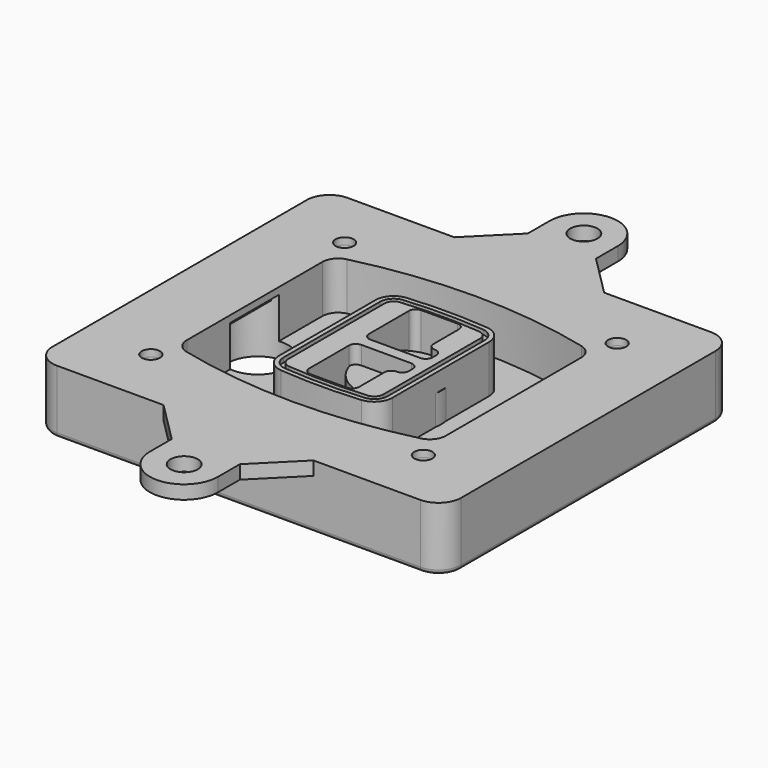
from build123d import *

# Parameters (mm, degrees)
F0_R      = 4
F1_DEPTH  = 25
F2_DEPTH  = 3
F3_DEPTH  = 18
F5_DEPTH  = 21
F6_DEPTH  = 2
F8_DEPTH  = 20
F9_DEPTH  = 16
F10_DEPTH = 25
F7_R      = 6
F7_R_2    = 4
F11_DEPTH = 6
F13_DEPTH = 9
F15_R     = 2
F16_R     = 4
F16_R_2   = 6
F17_DEPTH = 3


# Not quite as in the source:
# - a feature of the source that left no trace in its solid (it failed there, or was rolled back) is left out
# - a feature names something its author has since deleted; it is built from what else it names


with BuildPart() as f1:
    # F0 (on Top) → F1 (new body)
    with BuildSketch(Plane.XY):
        with BuildLine():
            ThreePointArc((-90, -70), (-87.0710678119, -77.0710678119), (-80, -80))
            Line((-80, -80), (80, -80))
            ThreePointArc((80, -80), (87.0710678119, -77.0710678119), (90, -70))
            Line((90, -70), (90, 70))
            ThreePointArc((90, 70), (87.0710678119, 77.0710678119), (80, 80))
            Line((80, 80), (-80, 80))
            ThreePointArc((-80, 80), (-87.0710678119, 77.0710678119), (-90, 70))
            Line((-90, 70), (-90, -70))
        make_face()
        with Locations((-60, -53.3333333333)):
            Circle(F0_R, mode=Mode.SUBTRACT)
        with Locations((60, -53.3333333333)):
            Circle(F0_R, mode=Mode.SUBTRACT)
        with Locations((-60, 53.3333333333)):
            Circle(F0_R, mode=Mode.SUBTRACT)
        with BuildLine():
            ThreePointArc((-64, 37.2990447398), (-61.0143011354, 45.9411029726), (-53.3306899286, 50.8970778549))
            ThreePointArc((-53.3306899286, 50.8970778549), (0, 57.3333333333), (53.3306899286, 50.8970778549))
            ThreePointArc((53.3306899286, 50.8970778549), (61.0143011354, 45.9411029726), (64, 37.2990447398))
            Line((64, 37.2990447398), (64, -37.2990447398))
            ThreePointArc((64, -37.2990447398), (61.0143011354, -45.9411029726), (53.3306899286, -50.8970778549))
            ThreePointArc((53.3306899286, -50.8970778549), (0, -57.3333333333), (-53.3306899286, -50.8970778549))
            ThreePointArc((-53.3306899286, -50.8970778549), (-61.0143011354, -45.9411029726), (-64, -37.2990447398))
            Line((-64, -37.2990447398), (-64, 37.2990447398))
        make_face(mode=Mode.SUBTRACT)
        with Locations((60, 53.3333333333)):
            Circle(F0_R, mode=Mode.SUBTRACT)
        with BuildLine():
            ThreePointArc((53.3306899286, 50.8970778549), (0, 57.3333333333), (-53.3306899286, 50.8970778549))
            ThreePointArc((-53.3306899286, 50.8970778549), (-61.0143011354, 45.9411029726), (-64, 37.2990447398))
            Line((-64, 37.2990447398), (-64, -37.2990447398))
            ThreePointArc((-64, -37.2990447398), (-61.0143011354, -45.9411029726), (-53.3306899286, -50.8970778549))
            ThreePointArc((-53.3306899286, -50.8970778549), (0, -57.3333333333), (53.3306899286, -50.8970778549))
            ThreePointArc((53.3306899286, -50.8970778549), (61.0143011354, -45.9411029726), (64, -37.2990447398))
            Line((64, -37.2990447398), (64, 37.2990447398))
            ThreePointArc((64, 37.2990447398), (61.0143011354, 45.9411029726), (53.3306899286, 50.8970778549))
        make_face()
        with BuildLine():
            Line((-60, -37.2990447398), (-60, 37.2990447398))
            ThreePointArc((-60, 37.2990447398), (-57.8673579538, 43.4719434775), (-52.3790642347, 47.0119255363))
            ThreePointArc((-52.3790642347, 47.0119255363), (0, 53.3333333333), (52.3790642347, 47.0119255363))
            ThreePointArc((52.3790642347, 47.0119255363), (57.8673579538, 43.4719434775), (60, 37.2990447398))
            Line((60, 37.2990447398), (60, -37.2990447398))
            ThreePointArc((60, -37.2990447398), (57.8673579538, -43.4719434775), (52.3790642347, -47.0119255363))
            ThreePointArc((52.3790642347, -47.0119255363), (0, -53.3333333333), (-52.3790642347, -47.0119255363))
            ThreePointArc((-52.3790642347, -47.0119255363), (-57.8673579538, -43.4719434775), (-60, -37.2990447398))
        make_face(mode=Mode.SUBTRACT)
        with BuildLine():
            ThreePointArc((-52.3790642347, 47.0119255363), (-57.8673579538, 43.4719434775), (-60, 37.2990447398))
            Line((-60, 37.2990447398), (-60, -37.2990447398))
            ThreePointArc((-60, -37.2990447398), (-57.8673579538, -43.4719434775), (-52.3790642347, -47.0119255363))
            ThreePointArc((-52.3790642347, -47.0119255363), (0, -53.3333333333), (52.3790642347, -47.0119255363))
            ThreePointArc((52.3790642347, -47.0119255363), (57.8673579538, -43.4719434775), (60, -37.2990447398))
            Line((60, -37.2990447398), (60, 37.2990447398))
            ThreePointArc((60, 37.2990447398), (57.8673579538, 43.4719434775), (52.3790642347, 47.0119255363))
            ThreePointArc((52.3790642347, 47.0119255363), (0, 53.3333333333), (-52.3790642347, 47.0119255363))
        make_face()
        with BuildLine():
            ThreePointArc((51.6653449643, 44.0980612973), (55.5071505677, 41.6200738562), (57, 37.2990447398))
            Line((57, 37.2990447398), (57, -37.2990447398))
            ThreePointArc((57, -37.2990447398), (55.5071505677, -41.6200738562), (51.6653449643, -44.0980612973))
            ThreePointArc((51.6653449643, -44.0980612973), (0, -50.3333333333), (-51.6653449643, -44.0980612973))
            ThreePointArc((-51.6653449643, -44.0980612973), (-55.5071505677, -41.6200738562), (-57, -37.2990447398))
            Line((-57, -37.2990447398), (-57, 37.2990447398))
            ThreePointArc((-57, 37.2990447398), (-55.5071505677, 41.6200738562), (-51.6653449643, 44.0980612973))
            ThreePointArc((-51.6653449643, 44.0980612973), (0, 50.3333333333), (51.6653449643, 44.0980612973))
        make_face(mode=Mode.SUBTRACT)
        with BuildLine():
            Line((57, -37.2990447398), (57, 37.2990447398))
            ThreePointArc((57, 37.2990447398), (55.5071505677, 41.6200738562), (51.6653449643, 44.0980612973))
            ThreePointArc((51.6653449643, 44.0980612973), (0, 50.3333333333), (-51.6653449643, 44.0980612973))
            ThreePointArc((-51.6653449643, 44.0980612973), (-55.5071505677, 41.6200738562), (-57, 37.2990447398))
            Line((-57, 37.2990447398), (-57, -37.2990447398))
            ThreePointArc((-57, -37.2990447398), (-55.5071505677, -41.6200738562), (-51.6653449643, -44.0980612973))
            ThreePointArc((-51.6653449643, -44.0980612973), (0, -50.3333333333), (51.6653449643, -44.0980612973))
            ThreePointArc((51.6653449643, -44.0980612973), (55.5071505677, -41.6200738562), (57, -37.2990447398))
        make_face()
    extrude(amount=-F1_DEPTH)

    # F0 (on Top) → F2 (join)
    with BuildSketch(Plane.XY):
        with BuildLine():
            ThreePointArc((-52.3790642347, 47.0119255363), (-57.8673579538, 43.4719434775), (-60, 37.2990447398))
            Line((-60, 37.2990447398), (-60, -37.2990447398))
            ThreePointArc((-60, -37.2990447398), (-57.8673579538, -43.4719434775), (-52.3790642347, -47.0119255363))
            ThreePointArc((-52.3790642347, -47.0119255363), (0, -53.3333333333), (52.3790642347, -47.0119255363))
            ThreePointArc((52.3790642347, -47.0119255363), (57.8673579538, -43.4719434775), (60, -37.2990447398))
            Line((60, -37.2990447398), (60, 37.2990447398))
            ThreePointArc((60, 37.2990447398), (57.8673579538, 43.4719434775), (52.3790642347, 47.0119255363))
            ThreePointArc((52.3790642347, 47.0119255363), (0, 53.3333333333), (-52.3790642347, 47.0119255363))
        make_face()
        with BuildLine():
            ThreePointArc((51.6653449643, 44.0980612973), (55.5071505677, 41.6200738562), (57, 37.2990447398))
            Line((57, 37.2990447398), (57, -37.2990447398))
            ThreePointArc((57, -37.2990447398), (55.5071505677, -41.6200738562), (51.6653449643, -44.0980612973))
            ThreePointArc((51.6653449643, -44.0980612973), (0, -50.3333333333), (-51.6653449643, -44.0980612973))
            ThreePointArc((-51.6653449643, -44.0980612973), (-55.5071505677, -41.6200738562), (-57, -37.2990447398))
            Line((-57, -37.2990447398), (-57, 37.2990447398))
            ThreePointArc((-57, 37.2990447398), (-55.5071505677, 41.6200738562), (-51.6653449643, 44.0980612973))
            ThreePointArc((-51.6653449643, 44.0980612973), (0, 50.3333333333), (51.6653449643, 44.0980612973))
        make_face(mode=Mode.SUBTRACT)
    extrude(amount=F2_DEPTH)

    # F0 (on Top) → F3 (cut)
    with BuildSketch(Plane.XY):
        with BuildLine():
            Line((57, -37.2990447398), (57, 37.2990447398))
            ThreePointArc((57, 37.2990447398), (55.5071505677, 41.6200738562), (51.6653449643, 44.0980612973))
            ThreePointArc((51.6653449643, 44.0980612973), (0, 50.3333333333), (-51.6653449643, 44.0980612973))
            ThreePointArc((-51.6653449643, 44.0980612973), (-55.5071505677, 41.6200738562), (-57, 37.2990447398))
            Line((-57, 37.2990447398), (-57, -37.2990447398))
            ThreePointArc((-57, -37.2990447398), (-55.5071505677, -41.6200738562), (-51.6653449643, -44.0980612973))
            ThreePointArc((-51.6653449643, -44.0980612973), (0, -50.3333333333), (51.6653449643, -44.0980612973))
            ThreePointArc((51.6653449643, -44.0980612973), (55.5071505677, -41.6200738562), (57, -37.2990447398))
        make_face()
    extrude(amount=-F3_DEPTH, mode=Mode.SUBTRACT)

    # F4 (on face) → F5 (join, through all)
    with BuildSketch(Plane.XY.offset(3)):
        with BuildLine():
            ThreePointArc((-25, -26.587695628), (-22.8992979869, -31.9912392117), (-17.7004291845, -34.5569740744))
            ThreePointArc((-17.7004291845, -34.5569740744), (0, -35.3333333333), (17.7004291845, -34.5569740744))
            ThreePointArc((17.7004291845, -34.5569740744), (22.8992979869, -31.9912392117), (25, -26.587695628))
            Line((25, -26.587695628), (25, 26.587695628))
            ThreePointArc((25, 26.587695628), (22.8992979869, 31.9912392117), (17.7004291845, 34.5569740744))
            ThreePointArc((17.7004291845, 34.5569740744), (0, 35.3333333333), (-17.7004291845, 34.5569740744))
            ThreePointArc((-17.7004291845, 34.5569740744), (-22.8992979869, 31.9912392117), (-25, 26.587695628))
            Line((-25, 26.587695628), (-25, -26.587695628))
        make_face()
        with BuildLine():
            ThreePointArc((17.5253218884, 32.5646544628), (21.4244734902, 30.6403533158), (23, 26.587695628))
            Line((23, 26.587695628), (23, -26.587695628))
            ThreePointArc((23, -26.587695628), (21.4244734902, -30.6403533158), (17.5253218884, -32.5646544628))
            ThreePointArc((17.5253218884, -32.5646544628), (0, -33.3333333333), (-17.5253218884, -32.5646544628))
            ThreePointArc((-17.5253218884, -32.5646544628), (-21.4244734902, -30.6403533158), (-23, -26.587695628))
            Line((-23, -26.587695628), (-23, 26.587695628))
            ThreePointArc((-23, 26.587695628), (-21.4244734902, 30.6403533158), (-17.5253218884, 32.5646544628))
            ThreePointArc((-17.5253218884, 32.5646544628), (0, 33.3333333333), (17.5253218884, 32.5646544628))
        make_face(mode=Mode.SUBTRACT)
        with BuildLine():
            Line((23, -26.587695628), (23, 26.587695628))
            ThreePointArc((23, 26.587695628), (21.4244734902, 30.6403533158), (17.5253218884, 32.5646544628))
            ThreePointArc((17.5253218884, 32.5646544628), (0, 33.3333333333), (-17.5253218884, 32.5646544628))
            ThreePointArc((-17.5253218884, 32.5646544628), (-21.4244734902, 30.6403533158), (-23, 26.587695628))
            Line((-23, 26.587695628), (-23, -26.587695628))
            ThreePointArc((-23, -26.587695628), (-21.4244734902, -30.6403533158), (-17.5253218884, -32.5646544628))
            ThreePointArc((-17.5253218884, -32.5646544628), (0, -33.3333333333), (17.5253218884, -32.5646544628))
            ThreePointArc((17.5253218884, -32.5646544628), (21.4244734902, -30.6403533158), (23, -26.587695628))
        make_face()
        with BuildLine():
            ThreePointArc((17.3502145923, 30.5723348512), (19.9496489934, 29.2894674198), (21, 26.587695628))
            Line((21, 26.587695628), (21, -26.587695628))
            ThreePointArc((21, -26.587695628), (19.9496489934, -29.2894674198), (17.3502145923, -30.5723348512))
            ThreePointArc((17.3502145923, -30.5723348512), (0, -31.3333333333), (-17.3502145923, -30.5723348512))
            ThreePointArc((-17.3502145923, -30.5723348512), (-19.9496489934, -29.2894674198), (-21, -26.587695628))
            Line((-21, -26.587695628), (-21, 26.587695628))
            ThreePointArc((-21, 26.587695628), (-19.9496489934, 29.2894674198), (-17.3502145923, 30.5723348512))
            ThreePointArc((-17.3502145923, 30.5723348512), (0, 31.3333333333), (17.3502145923, 30.5723348512))
        make_face(mode=Mode.SUBTRACT)
        with BuildLine():
            Line((21, -26.587695628), (21, 26.587695628))
            ThreePointArc((21, 26.587695628), (19.9496489934, 29.2894674198), (17.3502145923, 30.5723348512))
            ThreePointArc((17.3502145923, 30.5723348512), (0, 31.3333333333), (-17.3502145923, 30.5723348512))
            ThreePointArc((-17.3502145923, 30.5723348512), (-19.9496489934, 29.2894674198), (-21, 26.587695628))
            Line((-21, 26.587695628), (-21, -26.587695628))
            ThreePointArc((-21, -26.587695628), (-19.9496489934, -29.2894674198), (-17.3502145923, -30.5723348512))
            ThreePointArc((-17.3502145923, -30.5723348512), (0, -31.3333333333), (17.3502145923, -30.5723348512))
            ThreePointArc((17.3502145923, -30.5723348512), (19.9496489934, -29.2894674198), (21, -26.587695628))
        make_face()
        with BuildLine():
            Line((-8, -2.5), (14, -2.5))
            ThreePointArc((14, -2.5), (16.1213203436, -3.3786796564), (17, -5.5))
            Line((17, -5.5), (17, -7.5))
            ThreePointArc((17, -7.5), (16.1213203436, -9.6213203436), (14, -10.5))
            ThreePointArc((14, -10.5), (11.8786796564, -11.3786796564), (11, -13.5))
            Line((11, -13.5), (11, -27.5))
            ThreePointArc((11, -27.5), (10.1213203436, -29.6213203436), (8, -30.5))
            Line((8, -30.5), (-8, -30.5))
            ThreePointArc((-8, -30.5), (-10.1213203436, -29.6213203436), (-11, -27.5))
            Line((-11, -27.5), (-11, -5.5))
            ThreePointArc((-11, -5.5), (-10.1213203436, -3.3786796564), (-8, -2.5))
        make_face(mode=Mode.SUBTRACT)
        with BuildLine():
            ThreePointArc((-8, 2.5), (-10.1213203436, 3.3786796564), (-11, 5.5))
            Line((-11, 5.5), (-11, 27.5))
            ThreePointArc((-11, 27.5), (-10.1213203436, 29.6213203436), (-8, 30.5))
            Line((-8, 30.5), (8, 30.5))
            ThreePointArc((8, 30.5), (10.1213203436, 29.6213203436), (11, 27.5))
            Line((11, 27.5), (11, 13.5))
            ThreePointArc((11, 13.5), (11.8786796564, 11.3786796564), (14, 10.5))
            ThreePointArc((14, 10.5), (16.1213203436, 9.6213203436), (17, 7.5))
            Line((17, 7.5), (17, 5.5))
            ThreePointArc((17, 5.5), (16.1213203436, 3.3786796564), (14, 2.5))
            Line((14, 2.5), (-8, 2.5))
        make_face(mode=Mode.SUBTRACT)
    extrude(amount=-F5_DEPTH)

    # F4 (on face) → F6 (cut)
    with BuildSketch(Plane.XY.offset(3)):
        with BuildLine():
            Line((23, -26.587695628), (23, 26.587695628))
            ThreePointArc((23, 26.587695628), (21.4244734902, 30.6403533158), (17.5253218884, 32.5646544628))
            ThreePointArc((17.5253218884, 32.5646544628), (0, 33.3333333333), (-17.5253218884, 32.5646544628))
            ThreePointArc((-17.5253218884, 32.5646544628), (-21.4244734902, 30.6403533158), (-23, 26.587695628))
            Line((-23, 26.587695628), (-23, -26.587695628))
            ThreePointArc((-23, -26.587695628), (-21.4244734902, -30.6403533158), (-17.5253218884, -32.5646544628))
            ThreePointArc((-17.5253218884, -32.5646544628), (0, -33.3333333333), (17.5253218884, -32.5646544628))
            ThreePointArc((17.5253218884, -32.5646544628), (21.4244734902, -30.6403533158), (23, -26.587695628))
        make_face()
        with BuildLine():
            ThreePointArc((17.3502145923, 30.5723348512), (19.9496489934, 29.2894674198), (21, 26.587695628))
            Line((21, 26.587695628), (21, -26.587695628))
            ThreePointArc((21, -26.587695628), (19.9496489934, -29.2894674198), (17.3502145923, -30.5723348512))
            ThreePointArc((17.3502145923, -30.5723348512), (0, -31.3333333333), (-17.3502145923, -30.5723348512))
            ThreePointArc((-17.3502145923, -30.5723348512), (-19.9496489934, -29.2894674198), (-21, -26.587695628))
            Line((-21, -26.587695628), (-21, 26.587695628))
            ThreePointArc((-21, 26.587695628), (-19.9496489934, 29.2894674198), (-17.3502145923, 30.5723348512))
            ThreePointArc((-17.3502145923, 30.5723348512), (0, 31.3333333333), (17.3502145923, 30.5723348512))
        make_face(mode=Mode.SUBTRACT)
    extrude(amount=-F6_DEPTH, mode=Mode.SUBTRACT)

    # F7 (on face) → F8 (join)
    with BuildSketch(Plane(origin=(0, 0, -25), x_dir=(1, 0, 0), z_dir=(0, 0, -1))):
        with BuildLine():
            ThreePointArc((-6.71157564, 0), (6.7567035675, 13.4682792075), (20.224982775, 0))
            Line((20.224982775, 0), (25.224982775, 0))
            ThreePointArc((25.224982775, 0), (6.7567035675, 18.4682792075), (-11.71157564, 0))
            Line((-11.71157564, 0), (-6.71157564, 0))
        make_face()
        with BuildLine():
            Line((-6.71157564, 0), (20.224982775, 0))
            ThreePointArc((20.224982775, 0), (6.7567035675, 13.4682792075), (-6.71157564, 0))
        make_face()
        with BuildLine():
            ThreePointArc((-6.71157564, 0), (6.7567035675, -13.4682792075), (20.224982775, 0))
            Line((20.224982775, 0), (-6.71157564, 0))
        make_face()
        with BuildLine():
            Line((25.224982775, 0), (20.224982775, 0))
            ThreePointArc((20.224982775, 0), (6.7567035675, -13.4682792075), (-6.71157564, 0))
            Line((-6.71157564, 0), (-11.71157564, 0))
            ThreePointArc((-11.71157564, 0), (6.7567035675, -18.4682792075), (25.224982775, 0))
        make_face()
    extrude(amount=-F8_DEPTH)

    # F7 (on face) → F9 (cut)
    with BuildSketch(Plane(origin=(0, 0, -25), x_dir=(1, 0, 0), z_dir=(0, 0, -1))):
        with BuildLine():
            Line((-6.71157564, 0), (20.224982775, 0))
            ThreePointArc((20.224982775, 0), (6.7567035675, 13.4682792075), (-6.71157564, 0))
        make_face()
        with BuildLine():
            ThreePointArc((-6.71157564, 0), (6.7567035675, -13.4682792075), (20.224982775, 0))
            Line((20.224982775, 0), (-6.71157564, 0))
        make_face()
    extrude(amount=-F9_DEPTH, mode=Mode.SUBTRACT)

    # F7 (on face) → F10 (cut)
    with BuildSketch(Plane(origin=(0, 0, -25), x_dir=(1, 0, 0), z_dir=(0, 0, -1))):
        with BuildLine():
            Line((-69.0318229325, 0), (-42.0952645175, 0))
            ThreePointArc((-42.0952645175, 0), (-55.563543725, 13.4682792075), (-69.0318229325, 0))
        make_face()
        with BuildLine():
            ThreePointArc((-69.0318229325, 0), (-55.563543725, -13.4682792075), (-42.0952645175, 0))
            Line((-42.0952645175, 0), (-69.0318229325, 0))
        make_face()
    extrude(amount=-F10_DEPTH, mode=Mode.SUBTRACT)

    # F7 (on face) → F11 (cut)
    with BuildSketch(Plane(origin=(0, 0, -25), x_dir=(1, 0, 0), z_dir=(0, 0, -1))):
        with Locations((60, -53.3333333333)):
            Circle(F7_R)
        with Locations((60, -53.3333333333)):
            Circle(F7_R_2, mode=Mode.SUBTRACT)
        with Locations((-60, -53.3333333333)):
            Circle(F7_R)
        with Locations((-60, -53.3333333333)):
            Circle(F7_R_2, mode=Mode.SUBTRACT)
        with Locations((-60, 53.3333333333)):
            Circle(F7_R)
        with Locations((-60, 53.3333333333)):
            Circle(F7_R_2, mode=Mode.SUBTRACT)
        with Locations((60, 53.3333333333)):
            Circle(F7_R)
        with Locations((60, 53.3333333333)):
            Circle(F7_R_2, mode=Mode.SUBTRACT)
    extrude(amount=-F11_DEPTH, mode=Mode.SUBTRACT)

    # F12 (on face) → F13 (cut, through all)
    with BuildSketch(Plane(origin=(0, 0, -9), x_dir=(1, 0, 0), z_dir=(0, 0, -1))):
        with BuildLine():
            ThreePointArc((20.224982775, 0), (20.1663399806, 1.2554664788), (19.9909222755, 2.5))
            Line((19.9909222755, 2.5), (14, 2.5))
            ThreePointArc((14, 2.5), (16.1213203436, 3.3786796564), (17, 5.5))
            Line((17, 5.5), (17, 7.5))
            ThreePointArc((17, 7.5), (16.1213203436, 9.6213203436), (14, 10.5))
            ThreePointArc((14, 10.5), (12.1627255951, 11.1284134507), (11.0951631559, 12.750384826))
            ThreePointArc((11.0951631559, 12.750384826), (11.0476113807, 12.7664660322), (11, 12.7823698976))
            Line((11, 12.7823698976), (11, -12.7823698976))
            ThreePointArc((11, -12.7823698976), (11.0476113807, -12.7664660322), (11.0951631559, -12.750384826))
            ThreePointArc((11.0951631559, -12.750384826), (12.1627255951, -11.1284134507), (14, -10.5))
            ThreePointArc((14, -10.5), (16.1213203436, -9.6213203436), (17, -7.5))
            Line((17, -7.5), (17, -5.5))
            ThreePointArc((17, -5.5), (16.1213203436, -3.3786796564), (14, -2.5))
            Line((14, -2.5), (19.9909222755, -2.5))
            ThreePointArc((19.9909222755, -2.5), (20.1663399806, -1.2554664788), (20.224982775, 0))
        make_face()
    extrude(amount=F13_DEPTH, mode=Mode.SUBTRACT)

    # F15
    f15_edges = [f1.edges().sort_by_distance(p)[0] for p in [
        (0, -80, -25),
        (-87.071068, -77.071068, -25),
        (-90, 0, -25),
        (-87.071068, 77.071068, -25),
        (87.071068, -77.071068, -25),
        (0, 80, -25),
        (90, 0, -25),
        (87.071068, 77.071068, -25),
    ]]
    fillet(f15_edges, radius=F15_R)

    # F16 (on face) → F17 (join, symmetric)
    with BuildSketch(Plane.XY):
        with BuildLine():
            Line((-33.0668874085, 80), (-80, 80))
            ThreePointArc((-80, 80), (-87.0710678119, 77.0710678119), (-90, 70))
            Line((-90, 70), (-90, -70))
            ThreePointArc((-90, -70), (-87.0710678119, -77.0710678119), (-80, -80))
            Line((-80, -80), (-33.0668874085, -80))
            Line((-33.0668874085, -80), (32.9331125915, -80))
            Line((32.9331125915, -80), (80, -80))
            ThreePointArc((80, -80), (87.0710678119, -77.0710678119), (90, -70))
            Line((90, -70), (90, 70))
            ThreePointArc((90, 70), (87.0710678119, 77.0710678119), (80, 80))
            Line((80, 80), (32.9331125915, 80))
            Line((32.9331125915, 80), (-33.0668874085, 80))
        make_face()
        with Locations((-60, -53.3333333333)):
            Circle(F16_R, mode=Mode.SUBTRACT)
        with Locations((60, -53.3333333333)):
            Circle(F16_R, mode=Mode.SUBTRACT)
        with Locations((-60, 53.3333333333)):
            Circle(F16_R, mode=Mode.SUBTRACT)
        with BuildLine():
            ThreePointArc((-52.3790642347, 47.0119255363), (0, 53.3333333333), (52.3790642347, 47.0119255363))
            ThreePointArc((52.3790642347, 47.0119255363), (57.8673579538, 43.4719434775), (60, 37.2990447398))
            Line((60, 37.2990447398), (60, -37.2990447398))
            ThreePointArc((60, -37.2990447398), (57.8673579538, -43.4719434775), (52.3790642347, -47.0119255363))
            ThreePointArc((52.3790642347, -47.0119255363), (0, -53.3333333333), (-52.3790642347, -47.0119255363))
            ThreePointArc((-52.3790642347, -47.0119255363), (-57.8673579538, -43.4719434775), (-60, -37.2990447398))
            Line((-60, -37.2990447398), (-60, 37.2990447398))
            ThreePointArc((-60, 37.2990447398), (-57.8673579538, 43.4719434775), (-52.3790642347, 47.0119255363))
        make_face(mode=Mode.SUBTRACT)
        with Locations((60, 53.3333333333)):
            Circle(F16_R, mode=Mode.SUBTRACT)
        with BuildLine():
            Line((-15.0668874085, 98), (-33.0668874085, 80))
            Line((-33.0668874085, 80), (32.9331125915, 80))
            Line((32.9331125915, 80), (14.9331125915, 98))
            Line((14.9331125915, 98), (14.9331125915, 110))
            ThreePointArc((14.9331125915, 110), (-0.0668874085, 125), (-15.0668874085, 110))
            Line((-15.0668874085, 110), (-15.0668874085, 98))
        make_face()
        with Locations((0, 110)):
            Circle(F16_R_2, mode=Mode.SUBTRACT)
        with BuildLine():
            Line((32.9331125915, -80), (-33.0668874085, -80))
            Line((-33.0668874085, -80), (-15.0668874085, -98))
            Line((-15.0668874085, -98), (-15.0668874085, -110))
            ThreePointArc((-15.0668874085, -110), (-0.0668874085, -125), (14.9331125915, -110))
            Line((14.9331125915, -110), (14.9331125915, -98))
            Line((14.9331125915, -98), (32.9331125915, -80))
        make_face()
        with Locations((0, -110)):
            Circle(F16_R_2, mode=Mode.SUBTRACT)
    extrude(amount=F17_DEPTH, both=True)


solid = f1.part
